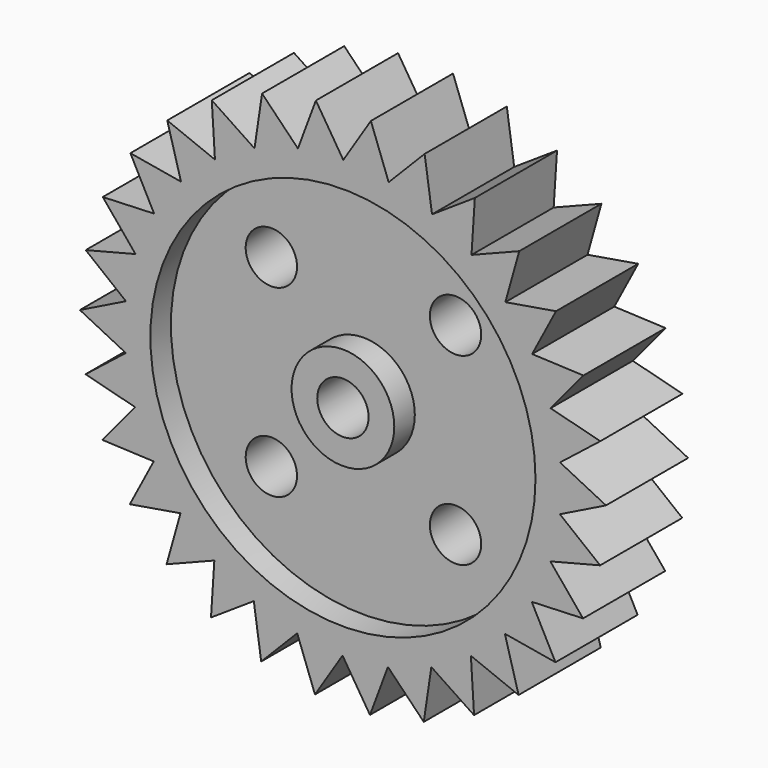
from build123d import *

# Parameters (mm, degrees)
F0_R            = 13.49375
F1_DEPTH        = 3.175
F3_DEPTH        = 6.35
F3_COPIES_COUNT = 30
F4_R            = 11.90625
F5_DEPTH        = 1.5875
F6_R            = 11.90625
F7_DEPTH        = 1.5875
F8_R            = 1.5875
F9_DEPTH        = 4.7635
F9_COPIES_COUNT = 4
F10_R           = 3.175
F11_DEPTH       = 1.5875
F12_R           = 3.175
F13_DEPTH       = 1.5875
F14_R           = 1.5875
F15_DEPTH       = 6.351


# Not quite as in the source:
# - a pattern or mirror of a feature is missing from the dataset's text; its kind, count and spacing are read off the source's solid


with BuildPart() as f1:
    # F0 (on Front) → F1 (new body, symmetric)
    with BuildSketch(Plane.XZ):
        Circle(F0_R)
    extrude(amount=F1_DEPTH, both=True)

    # F2 (on face) → F3 (join)
    with BuildSketch(Plane.XZ.offset(3.175)):
        with BuildLine():
            Line((1.7281408885, 16.1722566911), (0.0234068474, 13.4937296987))
            ThreePointArc((0.0234068474, 13.4937296987), (1.4337574514, 13.4173629538), (2.8283995087, 13.1939927725))
            Line((2.8283995087, 13.1939927725), (1.7281408885, 16.1722566911))
        make_face()
    f3 = extrude(amount=-F3_DEPTH)

    # F3_copies: F3 ×30 about axis
    f3_copies_axis = Axis((0, 0, 0), (0, 1, 0))
    for i in range(1, F3_COPIES_COUNT):
        add(f3.rotate(f3_copies_axis, i * 360 / F3_COPIES_COUNT))

    # F4 (on face) → F5 (cut)
    with BuildSketch(Plane.XZ.offset(3.175)):
        Circle(F4_R)
    extrude(amount=-F5_DEPTH, mode=Mode.SUBTRACT)

    # F6 (on face) → F7 (cut)
    with BuildSketch(Plane(origin=(0, 3.175, 0), x_dir=(-1, 0, 0), z_dir=(0, 1, 0))):
        Circle(F6_R)
    extrude(amount=-F7_DEPTH, mode=Mode.SUBTRACT)

    # F8 (on face) → F9 (cut, through all)
    with BuildSketch(Plane.XZ.offset(1.5875)):
        with Locations((-5.6939616362, 5.6939616362)):
            Circle(F8_R)
    f9 = extrude(amount=-F9_DEPTH, mode=Mode.SUBTRACT)

    # F9_copies: F9 ×4 about axis
    f9_copies_axis = Axis((0, 0, 0), (0, 1, 0))
    for i in range(1, F9_COPIES_COUNT):
        add(f9.rotate(f9_copies_axis, i * 360 / F9_COPIES_COUNT), mode=Mode.SUBTRACT)

    # F10 (on face) → F11 (join)
    with BuildSketch(Plane.XZ.offset(1.5875)):
        Circle(F10_R)
    extrude(amount=F11_DEPTH)

    # F12 (on face) → F13 (join)
    with BuildSketch(Plane(origin=(0, 1.5875, 0), x_dir=(-1, 0, 0), z_dir=(0, 1, 0))):
        Circle(F12_R)
    extrude(amount=F13_DEPTH)

    # F14 (on face) → F15 (cut, through all)
    with BuildSketch(Plane(origin=(0, 3.175, 0), x_dir=(-1, 0, 0), z_dir=(0, 1, 0))):
        Circle(F14_R)
    extrude(amount=-F15_DEPTH, mode=Mode.SUBTRACT)


solid = f1.part
